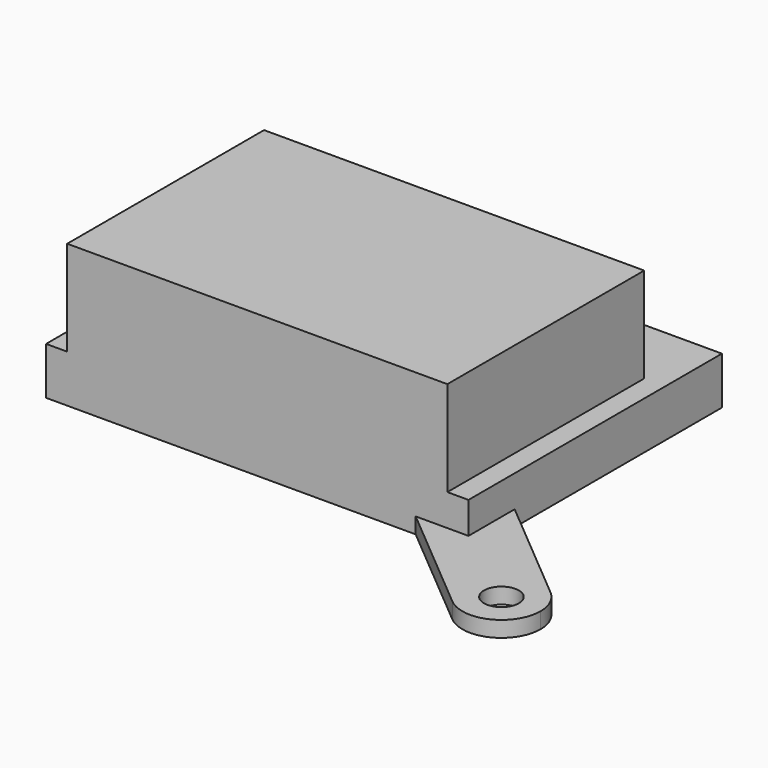
from build123d import *
from build123d import SkipClean  # not in build123d's __all__

# Parameters (mm, degrees)
F0_R      = 1.65
F1_DEPTH  = 1.5
F3_DEPTH  = 1.501
F4_DEPTH  = 1.5
F5_W      = 40
F5_H      = 30
F6_DEPTH  = 3
F7_W      = 36
F7_H      = 23.3
F8_DEPTH  = 9
F10_DEPTH = 1.501


with BuildPart() as f1:
    # F0 (on Top) → F1 (new body)
    with BuildSketch(Plane.XY):
        with BuildLine():
            ThreePointArc((-0.73370891, 14), (-0.4891889552, 6.9935887205), (0, 0))
            Line((0, 0), (65, 0))
            ThreePointArc((65, 0), (65.4891889552, 6.9935887205), (65.73370891, 14))
            ThreePointArc((65.73370891, 14), (65.7334108185, 21.0021379582), (65.488741818, 28))
            Line((65.488741818, 28), (57.299411547, 50.5))
            ThreePointArc((57.299411547, 50.5), (32.5, 63.5), (7.700588453, 50.5))
            Line((7.700588453, 50.5), (-0.488741818, 28))
            ThreePointArc((-0.488741818, 28), (-0.7334108185, 21.0021379582), (-0.73370891, 14))
        make_face()
        with Locations((4.5, 12.5)):
            Circle(F0_R, mode=Mode.SUBTRACT)
        with Locations((60.5, 12.5)):
            Circle(F0_R, mode=Mode.SUBTRACT)
        with Locations((15, 54.5)):
            Circle(F0_R, mode=Mode.SUBTRACT)
    extrude(amount=F1_DEPTH)

    # F2 (on face) → F3 (cut, through all)
    with BuildSketch(Plane.XY.offset(1.5)):
        with BuildLine():
            ThreePointArc((15.3946260476, 58.178895253), (17.4713893755, 57.2535857631), (18.6149922575, 55.2885626028))
            Line((18.6149922575, 55.2885626028), (20.0740134556, 48.6))
            Line((20.0740134556, 48.6), (52.5, 48.6))
            Line((52.5, 48.6), (52.5, 24.064025175))
            Line((52.5, 24.064025175), (62.8817094627, 15.3315119698))
            ThreePointArc((62.8817094627, 15.3315119698), (63.8542752579, 14.0616777817), (64.2, 12.5))
            ThreePointArc((64.2, 12.5), (62.0616777817, 9.1457247421), (58.1182905373, 9.6684880302))
            Line((58.1182905373, 9.6684880302), (47.5, 18.6))
            Line((47.5, 18.6), (17.5, 18.6))
            Line((17.5, 18.6), (6.8817094627, 9.6684880302))
            ThreePointArc((6.8817094627, 9.6684880302), (1.6684880302, 10.1182905373), (2.1182905373, 15.3315119698))
            Line((2.1182905373, 15.3315119698), (12.5, 24.064025175))
            Line((12.5, 24.064025175), (12.5, 48.6))
            Line((12.5, 48.6), (11.3850077425, 53.7114373972))
            ThreePointArc((11.3850077425, 53.7114373972), (11.308192582, 54.2539146721), (11.3123280961, 54.8017878876))
            ThreePointArc((11.3123280961, 54.8017878876), (9.4060764304, 52.7351735725), (7.700588453, 50.5))
            Line((7.700588453, 50.5), (-0.488741818, 28))
            ThreePointArc((-0.488741818, 28), (-0.733560046, 13.9914611719), (0, 0))
            Line((0, 0), (65, 0))
            ThreePointArc((65, 0), (65.733560046, 13.9914611719), (65.488741818, 28))
            Line((65.488741818, 28), (57.299411547, 50.5))
            ThreePointArc((57.299411547, 50.5), (37.9351551683, 63.0061258111), (15.3946260476, 58.178895253))
        make_face()
    extrude(amount=-F3_DEPTH, mode=Mode.SUBTRACT)

    # F2 (on face) → F4 (join)
    with BuildSketch(Plane.XY.offset(1.5)):
        with BuildLine():
            ThreePointArc((11.3123280961, 54.8017878876), (13.2791635515, 56.5801728664), (15.3946260476, 58.178895253))
            ThreePointArc((15.3946260476, 58.178895253), (12.6415574435, 57.3509206772), (11.3123280961, 54.8017878876))
        make_face()
    with SkipClean():  # cleaning this boolean's faces spoils the solid; the shape is the same uncleaned
        extrude(amount=-F4_DEPTH)

    # F5 (on face) → F6 (join)
    with BuildSketch(Plane.XY.offset(1.5)):
        with Locations((32.5, 33.6)):
            Rectangle(F5_W, F5_H)
    extrude(amount=F6_DEPTH)

    # F7 (on face) → F8 (join)
    with BuildSketch(Plane.XY.offset(4.5)):
        with Locations((32.5, 30.25)):
            Rectangle(F7_W, F7_H)
    extrude(amount=F8_DEPTH)

    # F9 (on face) → F10 (cut, through all)
    with BuildSketch(Plane.XY.offset(1.5)):
        with BuildLine():
            ThreePointArc((7.348777143, 10.0613592332), (8.0174859123, 11.2000796728), (8.25, 12.5))
            ThreePointArc((8.25, 12.5), (6.3550732217, 15.7590187699), (2.5853582175, 15.7243831727))
            ThreePointArc((2.5853582175, 15.7243831727), (1.6302243549, 10.0861052742), (7.348777143, 10.0613592332))
        make_face()
        with BuildLine():
            ThreePointArc((2.5853582175, 15.7243831727), (6.3550732217, 15.7590187699), (8.25, 12.5))
            ThreePointArc((8.25, 12.5), (8.0174859123, 11.2000796728), (7.348777143, 10.0613592332))
            Line((7.348777143, 10.0613592332), (17.5, 18.6))
            Line((17.5, 18.6), (12.5, 18.6))
            Line((12.5, 18.6), (12.5, 24.064025175))
            Line((12.5, 24.064025175), (2.5853582175, 15.7243831727))
        make_face()
    extrude(amount=-F10_DEPTH, mode=Mode.SUBTRACT)


solid = f1.part
